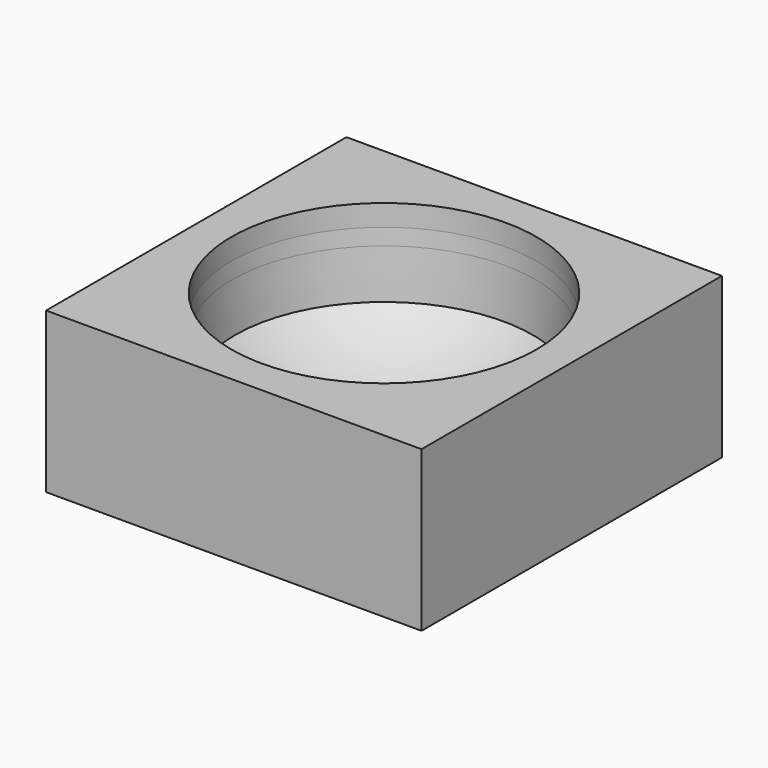
from build123d import *

# Parameters (mm, degrees)
F0_W     = 70.443585515
F0_H     = 70.443585515
F1_DEPTH = 30


# Not quite as in the source:
# - a feature names something its author has since deleted; it is built from what else it names


with BuildPart() as f1:
    # F0 (on Top) → F1 (new body)
    with BuildSketch(Plane.XY):
        Rectangle(F0_W, F0_H)
    extrude(amount=-F1_DEPTH)

    # F2 (on Front) → F3 (revolve, cut)
    with BuildSketch(Plane.XZ):
        with BuildLine():
            Line((0, -7), (0, -16))
            Line((0, -16), (0, -25.8))
            ThreePointArc((0, -25.8), (14.8091399143, -23.279001082), (27.95, -16))
            Line((27.95, -16), (28.45, -7))
            Line((28.45, -7), (28.6166666667, -4))
            Line((28.6166666667, -4), (28.6166666667, 0))
            Line((28.6166666667, 0), (0, 0))
            Line((0, 0), (0, -4))
            Line((0, -4), (0, -7))
        make_face()
    revolve(axis=Axis((0, 0, -11.5), (0, 0, 1)), mode=Mode.SUBTRACT)


solid = f1.part
